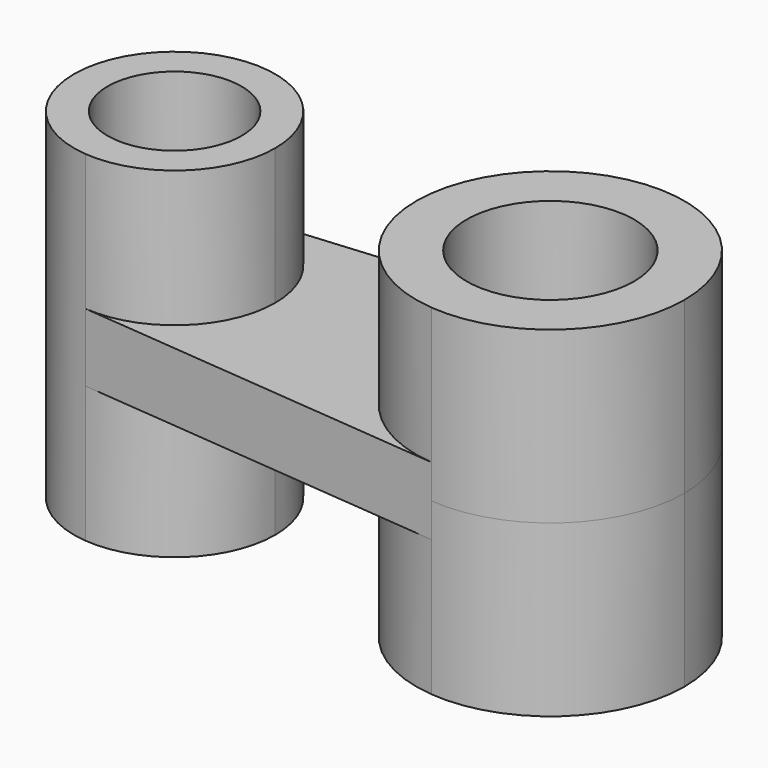
from build123d import *

# Parameters (mm, degrees)
F1_DEPTH      = 25.4
F1_DEPTH_BACK = 25.4
F2_DEPTH      = 5.08
F2_DEPTH_BACK = 5.08
F0_R          = 12.5
F3_DEPTH      = 25.4
F3_DEPTH_BACK = 25.4


# Not quite as in the source:
# - ends of sketch curves that miss each other by under 0.0002 mm in the source are joined


with BuildPart() as f1:
    # F0 (on Top) → F1 (new body, two sides)
    with BuildSketch(Plane.XY) as f1_sk:
        with BuildLine():
            ThreePointArc((-141.983922, -7.818031), (-146.8508026584, 3.2418013861), (-158.2932409879, 7.1247158622))
            ThreePointArc((-158.2932409879, 7.1247158622), (-168.0437543861, 2.3150883416), (-171.983922, -7.818031))
            ThreePointArc((-171.983922, -7.818031), (-168.0616462811, -17.9315874838), (-158.3460520332, -22.7560563639))
            ThreePointArc((-158.3460520332, -22.7560563639), (-146.8703655162, -18.8957552811), (-141.983922, -7.818031))
        make_face()
        with BuildLine():
            ThreePointArc((-146.983922, -7.818031), (-156.983922, -17.818031), (-166.983922, -7.818031))
            ThreePointArc((-166.983922, -7.818031), (-156.983922, 2.181969), (-146.983922, -7.818031))
        make_face(mode=Mode.SUBTRACT)
    extrude(amount=F1_DEPTH)
    extrude(f1_sk.sketch, amount=-F1_DEPTH_BACK)

    # F0 (on Top) → F2 (join, two sides)
    with BuildSketch(Plane.XY) as f2_sk:
        with BuildLine():
            ThreePointArc((-102.6737479638, -27.8325586075), (-120.8349111956, -7.8810440571), (-102.601594983, 12.004552808))
            Line((-102.601594983, 12.004552808), (-158.293241, 7.124716))
            ThreePointArc((-158.293241, 7.124716), (-146.8508026584, 3.2418013861), (-141.983922, -7.818031))
            ThreePointArc((-141.983922, -7.818031), (-146.8703655162, -18.8957552811), (-158.3460520332, -22.7560563639))
            Line((-158.3460520332, -22.7560563639), (-102.6737479638, -27.8325586075))
        make_face()
    extrude(amount=F2_DEPTH)
    extrude(f2_sk.sketch, amount=-F2_DEPTH_BACK)

    # F0 (on Top) → F3 (join, two sides)
    with BuildSketch(Plane.XY) as f3_sk:
        with BuildLine():
            ThreePointArc((-102.6737479638, -27.8325586075), (-87.3585958165, -22.6952258981), (-80.834944, -7.917268))
            ThreePointArc((-80.834944, -7.917268), (-87.3318521255, 6.8362573357), (-102.601594983, 12.004552808))
            ThreePointArc((-102.601594983, 12.004552808), (-120.8349111956, -7.8810440571), (-102.6737479638, -27.8325586075))
        make_face()
        with Locations((-100.834944, -7.917268)):
            Circle(F0_R, mode=Mode.SUBTRACT)
    extrude(amount=F3_DEPTH)
    extrude(f3_sk.sketch, amount=-F3_DEPTH_BACK)


solid = f1.part
